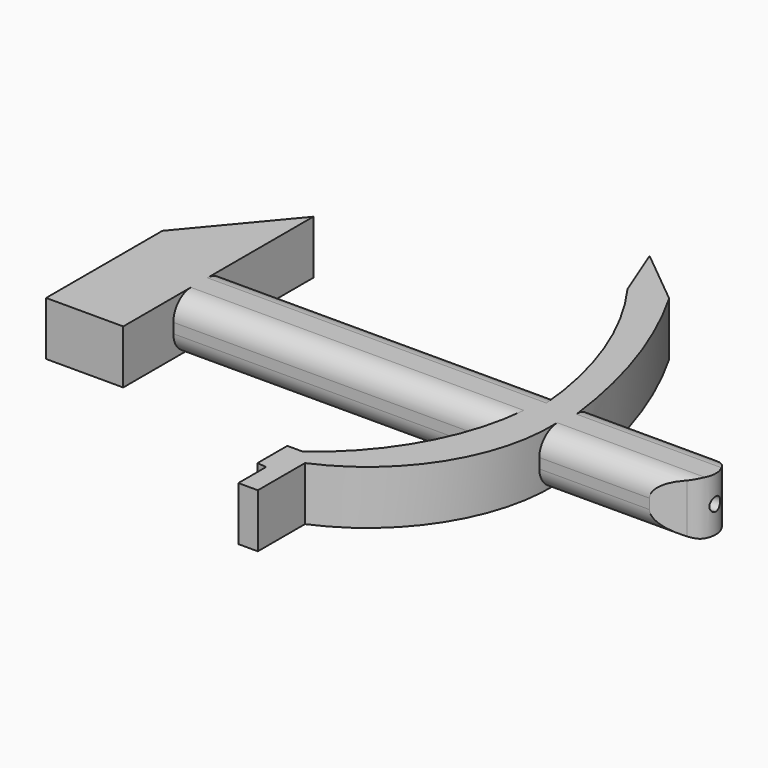
from build123d import *

# Parameters (mm, degrees)
F1_DEPTH    = 12.4968
F3_DEPTH    = 152.4
F4_T1_DEPTH = 61.7762374031
F5_R        = 5.08


# Not quite as in the source:
# - a fillet or chamfer that OpenCascade refuses, or shapes differently, is made with other operations: its cross-section is extruded or revolved along the edge and cut away or added
# - a feature names something its author has since deleted; it is built from what else it names


with BuildPart() as f1:
    # F0 (on Top) → F1 (new body)
    with BuildSketch(Plane.XY):
        with BuildLine():
            Line((-93.9849921167, 7.4851757918), (-16.1919427612, 7.4851757918))
            ThreePointArc((-16.1919427612, 7.4851757918), (-15.8959532901, 11.2229099464), (-15.7736930996, 14.9703515835))
            Line((-15.7736930996, 14.9703515835), (-93.9849921167, 14.9703515835))
            Line((-93.9849921167, 14.9703515835), (-93.9849921167, 7.4851757918))
        make_face()
        with BuildLine():
            Line((-93.9849921167, 0), (-17.3162451786, 0))
            ThreePointArc((-17.3162451786, 0), (-16.6663908007, 3.7294145399), (-16.1919427612, 7.4851757918))
            Line((-16.1919427612, 7.4851757918), (-93.9849921167, 7.4851757918))
            Line((-93.9849921167, 7.4851757918), (-93.9849921167, 0))
        make_face()
        Polygon((-93.9849921167, -14.5700745956), (-93.9849921167, 0), (-93.9849921167, 7.4851757918), (-93.9849921167, 14.9703515835), (-93.9849921167, 40.6753872946), (-111.9173921167, 19.2205523892), (-111.9173921167, 14.5700745956), (-111.9173921167, -14.5700745956), align=None)
        with BuildLine():
            Line((-15.7736930996, 14.9703515835), (-8.9203921167, 14.9703515835))
            ThreePointArc((-8.9203921167, 14.9703515835), (-14.3796310702, 36.1097695722), (-23.5038306564, 55.9447705746))
            Line((-23.5038306564, 55.9447705746), (-36.6789735854, 66.7365342379))
            Line((-36.6789735854, 66.7365342379), (-31.7310467362, 54.1373938322))
            ThreePointArc((-31.7310467362, 54.1373938322), (-21.3821676169, 35.5195355237), (-15.7736930996, 14.9703515835))
        make_face()
        with BuildLine():
            Line((-17.3162451786, 0), (-8.9203921167, 0))
            ThreePointArc((-8.9203921167, 0), (-8.270322019, 3.7175238692), (-8.0526666958, 7.4851757917))
            Line((-8.0526666958, 7.4851757918), (-16.1919427612, 7.4851757918))
            ThreePointArc((-16.1919427612, 7.4851757918), (-16.6663908007, 3.7294145399), (-17.3162451786, 0))
        make_face()
        with BuildLine():
            Line((-16.1919427612, 7.4851757918), (-8.0526666958, 7.4851757918))
            ThreePointArc((-8.0526666958, 7.4851757917), (-8.270322019, 11.2528277143), (-8.9203921167, 14.9703515835))
            Line((-8.9203921167, 14.9703515835), (-15.7736930996, 14.9703515835))
            ThreePointArc((-15.7736930996, 14.9703515835), (-15.8959532901, 11.2229099464), (-16.1919427612, 7.4851757918))
        make_face()
        with BuildLine():
            ThreePointArc((-34.6760861576, -35.9113998711), (-16.812117143, -21.5317519133), (-8.9203921167, 0))
            Line((-8.9203921167, 0), (-17.3162451786, 0))
            ThreePointArc((-17.3162451786, 0), (-24.4639001208, -18.231884723), (-37.7452522516, -32.6227247715))
            Line((-37.7452522516, -32.6227247715), (-41.4012260735, -32.6227247715))
            Line((-41.4012260735, -32.6227247715), (-41.4012260735, -41.2478148937))
            Line((-41.4012260735, -41.2478148937), (-39.2100475191, -41.5528100016))
            Line((-39.2100475191, -41.5528100016), (-39.2100475191, -49.5910942554))
            Line((-39.2100475191, -49.5910942554), (-34.6760861576, -49.5910942554))
            Line((-34.6760861576, -49.5910942554), (-34.6760861576, -35.9113998711))
        make_face()
        with BuildLine():
            ThreePointArc((-8.9203921167, 14.9703515835), (-8.270322019, 11.2528277143), (-8.0526666958, 7.4851757917))
            Line((-8.0526666958, 7.4851757918), (16.7025048286, 7.4851757918))
            Line((16.7025048286, 7.4851757918), (16.7025048286, 14.9703515835))
            Line((16.7025048286, 14.9703515835), (-8.9203921167, 14.9703515835))
        make_face()
        with BuildLine():
            ThreePointArc((-8.0526666958, 7.4851757917), (-8.270322019, 3.7175238692), (-8.9203921167, 0))
            Line((-8.9203921167, 0), (16.7025048286, 0))
            Line((16.7025048286, 0), (16.7025048286, 7.4851757918))
            Line((16.7025048286, 7.4851757918), (-8.0526666958, 7.4851757918))
        make_face()
        Polygon((16.7025048286, 7.4851757918), (16.7025048286, 0), (33.5264503956, 7.4851757918), (16.7025048286, 14.9703515835), align=None)
    extrude(amount=F1_DEPTH)

    # F2 (on face) → F3 (cut)
    with BuildSketch(Plane(origin=(-111.9173921167, 0, 0), x_dir=(0, -1, 0), z_dir=(-1, 0, 0))):
        with BuildLine():
            ThreePointArc((-5.9230757918, 6.2484), (-6.3806042889, 7.3529715029), (-7.4851757918, 7.8105))
            Line((-7.4851757918, 7.8105), (-7.4851757918, 4.6863))
            ThreePointArc((-7.4851757918, 4.6863), (-6.3806042889, 5.1438284971), (-5.9230757918, 6.2484))
        make_face()
        with BuildLine():
            Line((-7.4851757918, 4.6863), (-7.4851757918, 7.8105))
            ThreePointArc((-7.4851757918, 7.8105), (-9.0472757918, 6.2484), (-7.4851757918, 4.6863))
        make_face()
    extrude(amount=-F3_DEPTH, mode=Mode.SUBTRACT)

    # F4: fillet of radius 5.08 on 1 edges, made by hand

    # F4_s2 → F4_t1 (cut)
    with BuildSketch(Plane.XY.offset(-28.5449687015)):
        with BuildLine():
            ThreePointArc((23.0943727233, 2.843818927), (26.1093772139, 7.4851757918), (23.0943727233, 12.1265326565))
            Line((23.0943727233, 12.1265326565), (33.5264503956, 7.4851757918))
            Line((33.5264503956, 7.4851757918), (23.0943727233, 2.843818927))
        make_face()
    extrude(amount=F4_T1_DEPTH, mode=Mode.SUBTRACT)

    # F5
    f5_edges = [f1.edges().sort_by_distance(p)[0] for p in [
        (3.891056, 0, 12.4968),
        (3.891056, 14.970352, 12.4968),
        (3.891056, 0, 0),
        (3.891056, 14.970352, 0),
        (-54.879343, 14.970352, 12.4968),
        (-55.650619, 0, 12.4968),
        (-55.650619, 0, 0),
        (-54.879343, 14.970352, 0),
    ]]
    fillet(f5_edges, radius=F5_R)


solid = f1.part
